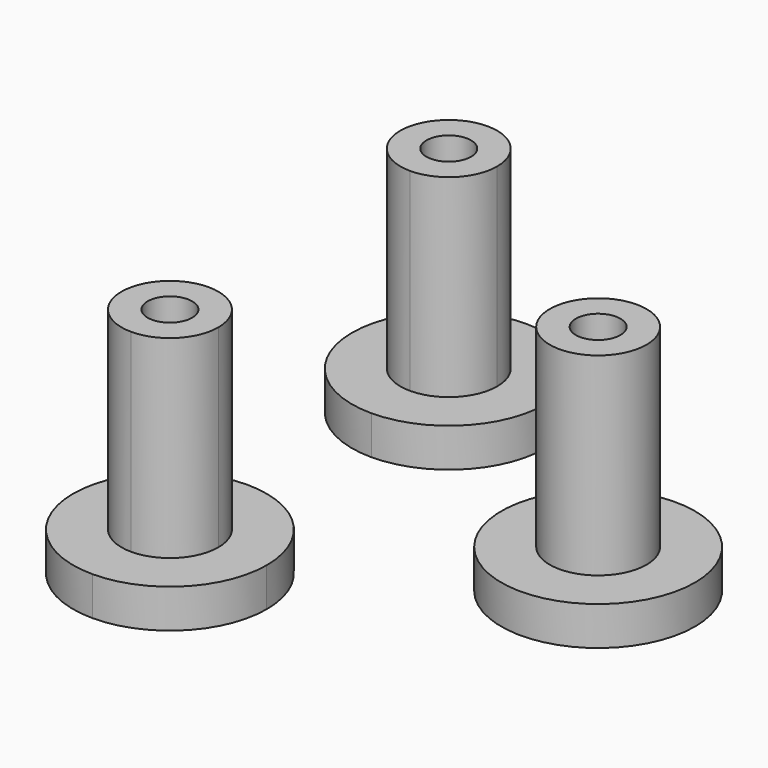
from build123d import *

# Parameters (mm, degrees)
F1_DEPTH = 2
F0_R     = 5
F0_R_2   = 2.5
F0_R_3   = 1.15
F2_DEPTH = 12


with BuildPart() as f1:
    # F0 (on Top) → F1 (new body)
    with BuildSketch(Plane.XY):
        with BuildLine():
            ThreePointArc((0, -4), (-5, -9), (0, -14))
            Line((0, -14), (0, -11.5))
            ThreePointArc((0, -11.5), (-2.5, -9), (0, -6.5))
            Line((0, -6.5), (0, -4))
        make_face()
        with BuildLine():
            Line((0, -11.5), (0, -14))
            ThreePointArc((0, -14), (3.5355339059, -12.5355339059), (5, -9))
            ThreePointArc((5, -9), (3.5355339059, -5.4644660941), (0, -4))
            Line((0, -4), (0, -6.5))
            ThreePointArc((0, -6.5), (1.767766953, -7.232233047), (2.5, -9))
            ThreePointArc((2.5, -9), (1.767766953, -10.767766953), (0, -11.5))
        make_face()
        with BuildLine():
            ThreePointArc((0, -6.5), (-2.5, -9), (0, -11.5))
            Line((0, -11.5), (0, -10.15))
            ThreePointArc((0, -10.15), (-1.15, -9), (0, -7.85))
            Line((0, -7.85), (0, -6.5))
        make_face()
        with BuildLine():
            Line((0, -10.15), (0, -11.5))
            ThreePointArc((0, -11.5), (1.767766953, -10.767766953), (2.5, -9))
            ThreePointArc((2.5, -9), (1.767766953, -7.232233047), (0, -6.5))
            Line((0, -6.5), (0, -7.85))
            ThreePointArc((0, -7.85), (0.8131727984, -8.1868272016), (1.15, -9))
            ThreePointArc((1.15, -9), (0.8131727984, -9.8131727984), (0, -10.15))
        make_face()
    extrude(amount=F1_DEPTH)

    # F0 (on Top) → F2 (join)
    with BuildSketch(Plane.XY):
        with BuildLine():
            ThreePointArc((0, -6.5), (-2.5, -9), (0, -11.5))
            Line((0, -11.5), (0, -10.15))
            ThreePointArc((0, -10.15), (-1.15, -9), (0, -7.85))
            Line((0, -7.85), (0, -6.5))
        make_face()
        with BuildLine():
            Line((0, -10.15), (0, -11.5))
            ThreePointArc((0, -11.5), (1.767766953, -10.767766953), (2.5, -9))
            ThreePointArc((2.5, -9), (1.767766953, -7.232233047), (0, -6.5))
            Line((0, -6.5), (0, -7.85))
            ThreePointArc((0, -7.85), (0.8131727984, -8.1868272016), (1.15, -9))
            ThreePointArc((1.15, -9), (0.8131727984, -9.8131727984), (0, -10.15))
        make_face()
    extrude(amount=F2_DEPTH)


with BuildPart() as f1b:
    # F0 (on Top) → F1, piece 2 (new body)
    with BuildSketch(Plane.XY):
        with BuildLine():
            ThreePointArc((0, 14), (-5, 9), (0, 4))
            Line((0, 4), (0, 6.5))
            ThreePointArc((0, 6.5), (-2.5, 9), (0, 11.5))
            Line((0, 11.5), (0, 14))
        make_face()
        with BuildLine():
            Line((0, 6.5), (0, 4))
            ThreePointArc((0, 4), (3.5355339059, 5.4644660941), (5, 9))
            ThreePointArc((5, 9), (3.5355339059, 12.5355339059), (0, 14))
            Line((0, 14), (0, 11.5))
            ThreePointArc((0, 11.5), (1.767766953, 10.767766953), (2.5, 9))
            ThreePointArc((2.5, 9), (1.767766953, 7.232233047), (0, 6.5))
        make_face()
        with BuildLine():
            ThreePointArc((0, 11.5), (-2.5, 9), (0, 6.5))
            Line((0, 6.5), (0, 7.85))
            ThreePointArc((0, 7.85), (-1.15, 9), (0, 10.15))
            Line((0, 10.15), (0, 11.5))
        make_face()
        with BuildLine():
            Line((0, 7.85), (0, 6.5))
            ThreePointArc((0, 6.5), (1.767766953, 7.232233047), (2.5, 9))
            ThreePointArc((2.5, 9), (1.767766953, 10.767766953), (0, 11.5))
            Line((0, 11.5), (0, 10.15))
            ThreePointArc((0, 10.15), (0.8131727984, 9.8131727984), (1.15, 9))
            ThreePointArc((1.15, 9), (0.8131727984, 8.1868272016), (0, 7.85))
        make_face()
    extrude(amount=F1_DEPTH)

    # F0 (on Top) → F2, piece 2 (join)
    with BuildSketch(Plane.XY):
        with BuildLine():
            ThreePointArc((0, 11.5), (-2.5, 9), (0, 6.5))
            Line((0, 6.5), (0, 7.85))
            ThreePointArc((0, 7.85), (-1.15, 9), (0, 10.15))
            Line((0, 10.15), (0, 11.5))
        make_face()
        with BuildLine():
            Line((0, 7.85), (0, 6.5))
            ThreePointArc((0, 6.5), (1.767766953, 7.232233047), (2.5, 9))
            ThreePointArc((2.5, 9), (1.767766953, 10.767766953), (0, 11.5))
            Line((0, 11.5), (0, 10.15))
            ThreePointArc((0, 10.15), (0.8131727984, 9.8131727984), (1.15, 9))
            ThreePointArc((1.15, 9), (0.8131727984, 8.1868272016), (0, 7.85))
        make_face()
    extrude(amount=F2_DEPTH)


with BuildPart() as f1c:
    # F0 (on Top) → F1, piece 3 (new body)
    with BuildSketch(Plane.XY):
        with Locations((14.4317867234, 0.602257438)):
            Circle(F0_R)
        with Locations((14.4317867234, 0.602257438)):
            Circle(F0_R_2, mode=Mode.SUBTRACT)
        with Locations((14.4317867234, 0.602257438)):
            Circle(F0_R_2)
        with Locations((14.4317867234, 0.602257438)):
            Circle(F0_R_3, mode=Mode.SUBTRACT)
    extrude(amount=F1_DEPTH)

    # F0 (on Top) → F2, piece 3 (join)
    with BuildSketch(Plane.XY):
        with Locations((14.4317867234, 0.602257438)):
            Circle(F0_R_2)
        with Locations((14.4317867234, 0.602257438)):
            Circle(F0_R_3, mode=Mode.SUBTRACT)
    extrude(amount=F2_DEPTH)


solid = Compound([f1.part, f1b.part, f1c.part])
